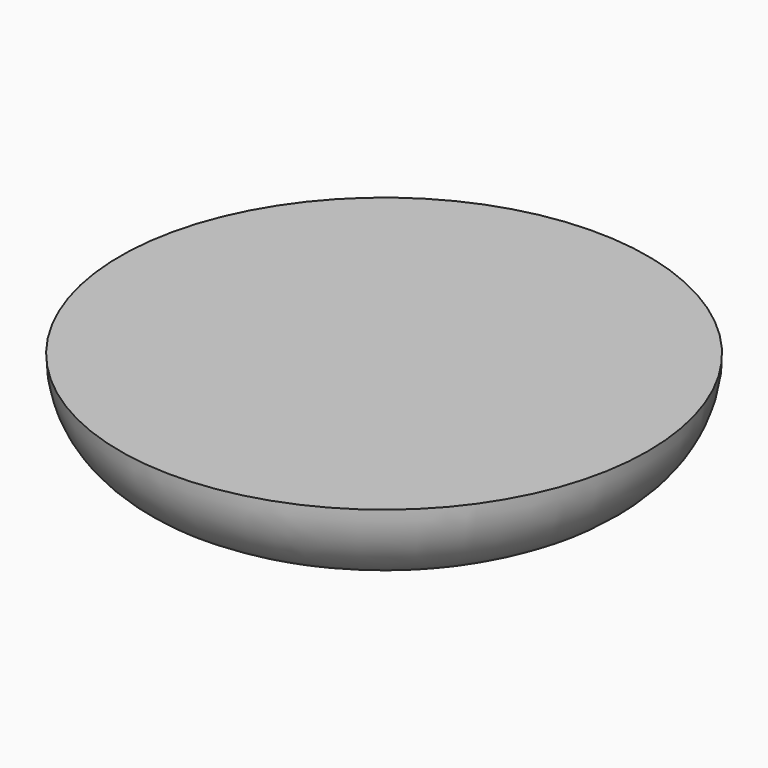
from build123d import *

# Parameters (mm, degrees)
F0_R     = 3
F1_DEPTH = 1
F2_R     = 0.99999


# Not quite as in the source:
# - a fillet or chamfer is up to 0.001 mm smaller than in the source, because OpenCascade refuses the exact size


with BuildPart() as f1:
    # F0 (on Top) → F1 (new body)
    with BuildSketch(Plane.XY):
        Circle(F0_R)
    extrude(amount=F1_DEPTH)

    # F2 (radius 1 in the source; OpenCascade refuses exactly that, so slightly less here)
    f2_edges = [f1.edges().sort_by_distance(p)[0] for p in [
        (-3, 0, 0),
    ]]
    fillet(f2_edges, radius=F2_R)


solid = f1.part
